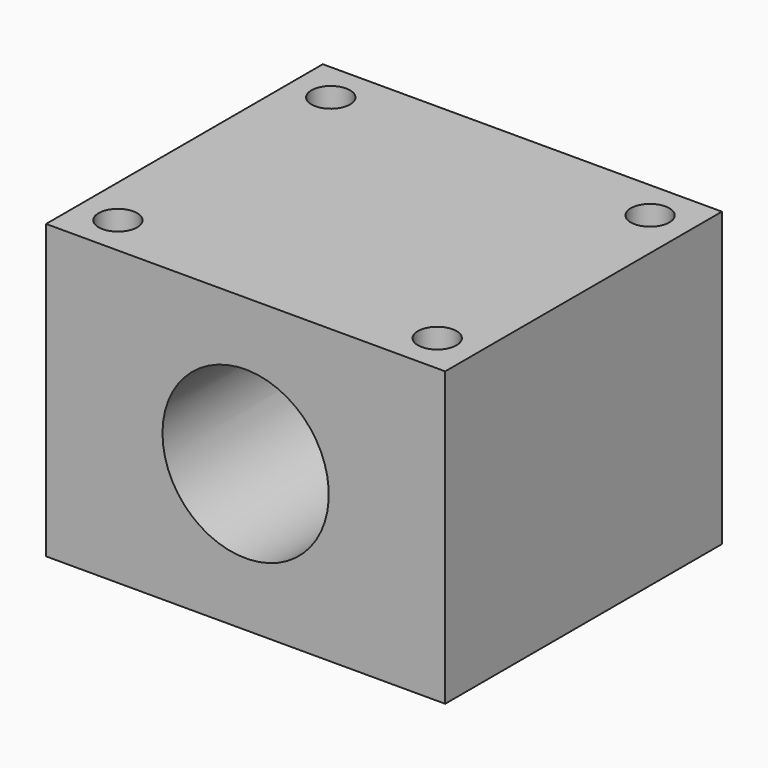
from build123d import *

# Parameters (mm, degrees)
F0_W     = 30
F0_H     = 26
F0_R     = 1.45
F1_DEPTH = 22
F2_R     = 6.25
F3_DEPTH = 26.001
F4_R     = 1.5
F5_DEPTH = 13


# Not quite as in the source:
# - a feature names something its author has since deleted; it is built from what else it names


with BuildPart() as f1:
    # F0 (on Top) → F1 (new body)
    with BuildSketch(Plane.XY):
        Rectangle(F0_W, F0_H)
        with Locations((-12, -10)):
            Circle(F0_R, mode=Mode.SUBTRACT)
        with Locations((12, -10)):
            Circle(F0_R, mode=Mode.SUBTRACT)
        with Locations((-12, 10)):
            Circle(F0_R, mode=Mode.SUBTRACT)
        with Locations((12, 10)):
            Circle(F0_R, mode=Mode.SUBTRACT)
    extrude(amount=F1_DEPTH)

    # F2 (on face) → F3 (cut, through all)
    with BuildSketch(Plane(origin=(0, 13, 0), x_dir=(-1, 0, 0), z_dir=(0, 1, 0))):
        with Locations((0, 11)):
            Circle(F2_R)
    extrude(amount=-F3_DEPTH, mode=Mode.SUBTRACT)

    # F4 (on face) → F5 (cut)
    with BuildSketch(Plane(origin=(-15, 0, 0), x_dir=(0, -1, 0), z_dir=(-1, 0, 0))):
        with Locations((0, 11)):
            Circle(F4_R)
    extrude(amount=-F5_DEPTH, mode=Mode.SUBTRACT)


solid = f1.part
